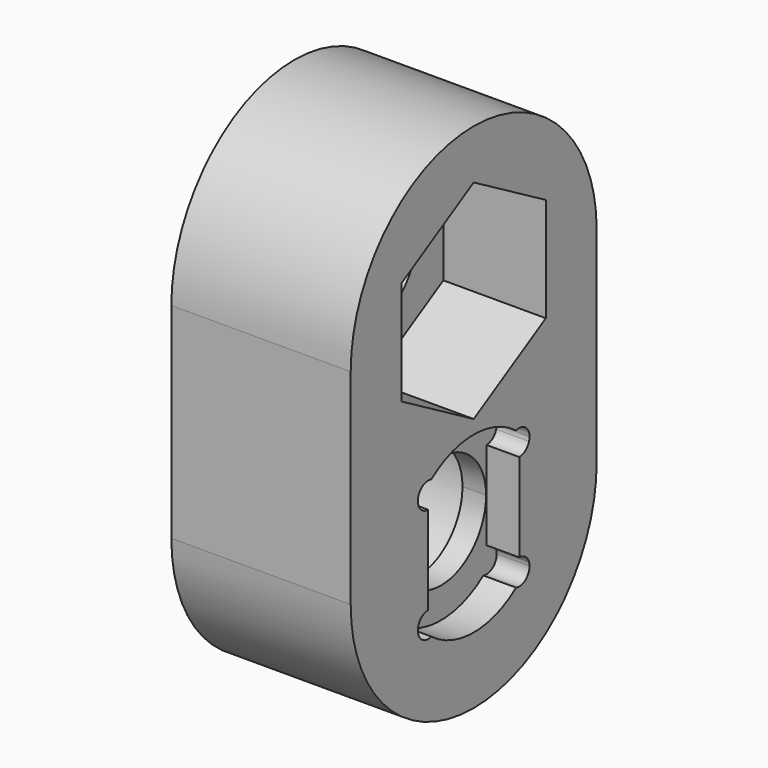
from build123d import *

# Parameters (mm, degrees)
F1_DEPTH = 5.55752
F2_R     = 1.75
F3_DEPTH = 1.016
F4_R     = 1.75
F5_DEPTH = 1.016
F6_DEPTH = 3.175
F7_R     = 2.667
F7_R_2   = 1.75
F8_DEPTH = 3.81


# Not quite as in the source:
# - a feature names something its author has since deleted; it is built from what else it names


with BuildPart() as f1:
    # F0 (on Right) → F1 (new body)
    with BuildSketch(Plane.YZ):
        with BuildLine():
            ThreePointArc((0.636344373, -4.7197957677), (2.2310225415, -4.2076055743), (3.5497579143, -3.175))
            ThreePointArc((3.5497579143, -3.175), (2.2310225415, -2.1423944257), (0.636344373, -1.6302042323))
            ThreePointArc((0.636344373, -1.6302042323), (0, -1.75), (-0.636344373, -1.6302042323))
            ThreePointArc((-0.636344373, -1.6302042323), (-2.2310225415, -2.1423944257), (-3.5497579143, -3.175))
            ThreePointArc((-3.5497579143, -3.175), (-2.2310225415, -4.2076055743), (-0.636344373, -4.7197957677))
            ThreePointArc((-0.636344373, -4.7197957677), (0, -4.6), (0.636344373, -4.7197957677))
        make_face()
        with BuildLine():
            ThreePointArc((3.5497579143, -3.175), (4.4489958596, -1.6993652025), (4.7625, 0))
            ThreePointArc((4.7625, 0), (0, 4.7625), (-4.7625, 0))
            ThreePointArc((-4.7625, 0), (-4.4489958596, -1.6993652025), (-3.5497579143, -3.175))
            ThreePointArc((-3.5497579143, -3.175), (-2.2310225415, -2.1423944257), (-0.636344373, -1.6302042323))
            ThreePointArc((-0.636344373, -1.6302042323), (-0.9871416685, 1.4450091094), (1.75, 0))
            ThreePointArc((1.75, 0), (1.4450091094, -0.9871416685), (0.636344373, -1.6302042323))
            ThreePointArc((0.636344373, -1.6302042323), (2.2310225415, -2.1423944257), (3.5497579143, -3.175))
        make_face()
        with BuildLine():
            Line((4.7625, -6.35), (4.7625, 0))
            ThreePointArc((4.7625, 0), (4.4489958596, -1.6993652025), (3.5497579143, -3.175))
            ThreePointArc((3.5497579143, -3.175), (4.4489958596, -4.6506347975), (4.7625, -6.35))
        make_face()
        with BuildLine():
            ThreePointArc((4.7625, -6.35), (4.4489958596, -4.6506347975), (3.5497579143, -3.175))
            ThreePointArc((3.5497579143, -3.175), (2.2310225415, -4.2076055743), (0.636344373, -4.7197957677))
            ThreePointArc((0.636344373, -4.7197957677), (1.4450091094, -5.3628583315), (1.75, -6.35))
            ThreePointArc((1.75, -6.35), (-0.9871416685, -7.7950091094), (-0.636344373, -4.7197957677))
            ThreePointArc((-0.636344373, -4.7197957677), (-2.2310225415, -4.2076055743), (-3.5497579143, -3.175))
            ThreePointArc((-3.5497579143, -3.175), (-4.4489958596, -4.6506347975), (-4.7625, -6.35))
            ThreePointArc((-4.7625, -6.35), (0, -11.1125), (4.7625, -6.35))
        make_face()
        with BuildLine():
            ThreePointArc((-3.5497579143, -3.175), (-4.4489958596, -1.6993652025), (-4.7625, 0))
            Line((-4.7625, 0), (-4.7625, -6.35))
            ThreePointArc((-4.7625, -6.35), (-4.4489958596, -4.6506347975), (-3.5497579143, -3.175))
        make_face()
    extrude(amount=F1_DEPTH)

    # F2 (on face) → F3 (cut)
    with BuildSketch(Plane.YZ.offset(5.55752)):
        with BuildLine():
            ThreePointArc((1.368425, -4.5847), (1.4846669962, -4.8653330038), (1.7653, -4.981575))
            Line((1.7653, -4.981575), (1.7653, -4.5847))
            Line((1.7653, -4.5847), (1.368425, -4.5847))
        make_face()
        with BuildLine():
            Line((1.7653, -4.5847), (1.7653, -4.981575))
            ThreePointArc((1.7653, -4.981575), (1.9986038099, -4.9057593371), (2.1427708235, -4.7072787218))
            ThreePointArc((2.1427708235, -4.7072787218), (1.9091883092, -4.4408116908), (1.6427212782, -4.2072291765))
            ThreePointArc((1.6427212782, -4.2072291765), (1.4442406629, -4.3513961901), (1.368425, -4.5847))
            Line((1.368425, -4.5847), (1.7653, -4.5847))
        make_face()
        with BuildLine():
            ThreePointArc((1.7653, -7.718425), (1.4846669962, -7.8346669962), (1.368425, -8.1153))
            Line((1.368425, -8.1153), (1.7653, -8.1153))
            Line((1.7653, -8.1153), (1.7653, -7.718425))
        make_face()
        with BuildLine():
            Line((1.7653, -8.1153), (1.368425, -8.1153))
            ThreePointArc((1.368425, -8.1153), (1.4442406629, -8.3486038099), (1.6427212782, -8.4927708235))
            ThreePointArc((1.6427212782, -8.4927708235), (1.9091883092, -8.2591883092), (2.1427708235, -7.9927212782))
            ThreePointArc((2.1427708235, -7.9927212782), (1.9986038099, -7.7942406629), (1.7653, -7.718425))
            Line((1.7653, -7.718425), (1.7653, -8.1153))
        make_face()
        with BuildLine():
            Line((-1.368425, -8.1153), (-1.7653, -8.1153))
            Line((-1.7653, -8.1153), (-1.7653, -7.718425))
            ThreePointArc((-1.7653, -7.718425), (-1.9986038099, -7.7942406629), (-2.1427708235, -7.9927212782))
            ThreePointArc((-2.1427708235, -7.9927212782), (-1.9091883092, -8.2591883092), (-1.6427212782, -8.4927708235))
            ThreePointArc((-1.6427212782, -8.4927708235), (-1.4442406629, -8.3486038099), (-1.368425, -8.1153))
        make_face()
        with BuildLine():
            Line((-1.7653, -7.718425), (-1.7653, -8.1153))
            Line((-1.7653, -8.1153), (-1.368425, -8.1153))
            ThreePointArc((-1.368425, -8.1153), (-1.4846669962, -7.8346669962), (-1.7653, -7.718425))
        make_face()
        with BuildLine():
            Line((-1.7653, -4.5847), (-1.7653, -4.981575))
            ThreePointArc((-1.7653, -4.981575), (-1.4846669962, -4.8653330038), (-1.368425, -4.5847))
            Line((-1.368425, -4.5847), (-1.7653, -4.5847))
        make_face()
        with BuildLine():
            ThreePointArc((-2.1427708235, -4.7072787218), (-1.9986038099, -4.9057593371), (-1.7653, -4.981575))
            Line((-1.7653, -4.981575), (-1.7653, -4.5847))
            Line((-1.7653, -4.5847), (-1.368425, -4.5847))
            ThreePointArc((-1.368425, -4.5847), (-1.4442406629, -4.3513961901), (-1.6427212782, -4.2072291765))
            ThreePointArc((-1.6427212782, -4.2072291765), (-1.9091883092, -4.4408116908), (-2.1427708235, -4.7072787218))
        make_face()
        with BuildLine():
            ThreePointArc((-1.7653, -7.718425), (-1.4846669962, -7.8346669962), (-1.368425, -8.1153))
            Line((-1.368425, -8.1153), (1.368425, -8.1153))
            ThreePointArc((1.368425, -8.1153), (1.4846669962, -7.8346669962), (1.7653, -7.718425))
            Line((1.7653, -7.718425), (1.7653, -4.981575))
            ThreePointArc((1.7653, -4.981575), (1.4846669962, -4.8653330038), (1.368425, -4.5847))
            Line((1.368425, -4.5847), (-1.368425, -4.5847))
            ThreePointArc((-1.368425, -4.5847), (-1.4846669962, -4.8653330038), (-1.7653, -4.981575))
            Line((-1.7653, -4.981575), (-1.7653, -7.718425))
        make_face()
        with Locations((0, -6.35)):
            Circle(F2_R, mode=Mode.SUBTRACT)
        with BuildLine():
            ThreePointArc((-1.6427212782, -4.2072291765), (-2.0459330038, -4.3040669962), (-2.1427708235, -4.7072787218))
            ThreePointArc((-2.1427708235, -4.7072787218), (-1.9091883092, -4.4408116908), (-1.6427212782, -4.2072291765))
        make_face()
        with BuildLine():
            ThreePointArc((1.6427212782, -4.2072291765), (1.9091883092, -4.4408116908), (2.1427708235, -4.7072787218))
            ThreePointArc((2.1427708235, -4.7072787218), (2.1572939405, -4.6467525283), (2.162175, -4.5847))
            ThreePointArc((2.162175, -4.5847), (1.9986038099, -4.2636406629), (1.6427212782, -4.2072291765))
        make_face()
        with BuildLine():
            ThreePointArc((2.1427708235, -7.9927212782), (1.9091883092, -8.2591883092), (1.6427212782, -8.4927708235))
            ThreePointArc((1.6427212782, -8.4927708235), (1.9986038099, -8.4363593371), (2.162175, -8.1153))
            ThreePointArc((2.162175, -8.1153), (2.1572939405, -8.0532474717), (2.1427708235, -7.9927212782))
        make_face()
        with BuildLine():
            ThreePointArc((-2.1427708235, -7.9927212782), (-2.0459330038, -8.3959330038), (-1.6427212782, -8.4927708235))
            ThreePointArc((-1.6427212782, -8.4927708235), (-1.9091883092, -8.2591883092), (-2.1427708235, -7.9927212782))
        make_face()
        with BuildLine():
            ThreePointArc((-1.6427212782, -4.2072291765), (-1.4442406629, -4.3513961901), (-1.368425, -4.5847))
            Line((-1.368425, -4.5847), (1.368425, -4.5847))
            ThreePointArc((1.368425, -4.5847), (1.4442406629, -4.3513961901), (1.6427212782, -4.2072291765))
            ThreePointArc((1.6427212782, -4.2072291765), (0, -3.65), (-1.6427212782, -4.2072291765))
        make_face()
        with BuildLine():
            Line((1.368425, -8.1153), (-1.368425, -8.1153))
            ThreePointArc((-1.368425, -8.1153), (-1.4442406629, -8.3486038099), (-1.6427212782, -8.4927708235))
            ThreePointArc((-1.6427212782, -8.4927708235), (0, -9.05), (1.6427212782, -8.4927708235))
            ThreePointArc((1.6427212782, -8.4927708235), (1.4442406629, -8.3486038099), (1.368425, -8.1153))
        make_face()
    extrude(amount=-F3_DEPTH, mode=Mode.SUBTRACT)

    # F4 (on face) → F5 (cut)
    with BuildSketch(Plane(origin=(0, 0, 0), x_dir=(0, -1, 0), z_dir=(-1, 0, 0))):
        with BuildLine():
            ThreePointArc((1.7653, -1.368425), (1.4846669962, -1.4846669962), (1.368425, -1.7653))
            Line((1.368425, -1.7653), (1.7653, -1.7653))
            Line((1.7653, -1.7653), (1.7653, -1.368425))
        make_face()
        with BuildLine():
            Line((1.7653, -1.7653), (1.368425, -1.7653))
            ThreePointArc((1.368425, -1.7653), (1.4442406629, -1.9986038099), (1.6427212782, -2.1427708235))
            ThreePointArc((1.6427212782, -2.1427708235), (1.9091883092, -1.9091883092), (2.1427708235, -1.6427212782))
            ThreePointArc((2.1427708235, -1.6427212782), (1.9986038099, -1.4442406629), (1.7653, -1.368425))
            Line((1.7653, -1.368425), (1.7653, -1.7653))
        make_face()
        with BuildLine():
            Line((-1.7653, -1.368425), (-1.7653, -1.7653))
            Line((-1.7653, -1.7653), (-1.368425, -1.7653))
            ThreePointArc((-1.368425, -1.7653), (-1.4846669962, -1.4846669962), (-1.7653, -1.368425))
        make_face()
        with BuildLine():
            Line((-1.368425, -1.7653), (-1.7653, -1.7653))
            Line((-1.7653, -1.7653), (-1.7653, -1.368425))
            ThreePointArc((-1.7653, -1.368425), (-1.9986038099, -1.4442406629), (-2.1427708235, -1.6427212782))
            ThreePointArc((-2.1427708235, -1.6427212782), (-1.9091883092, -1.9091883092), (-1.6427212782, -2.1427708235))
            ThreePointArc((-1.6427212782, -2.1427708235), (-1.4442406629, -1.9986038099), (-1.368425, -1.7653))
        make_face()
        with BuildLine():
            Line((-1.7653, 1.7653), (-1.7653, 1.368425))
            ThreePointArc((-1.7653, 1.368425), (-1.4846669962, 1.4846669962), (-1.368425, 1.7653))
            Line((-1.368425, 1.7653), (-1.7653, 1.7653))
        make_face()
        with BuildLine():
            ThreePointArc((-2.1427708235, 1.6427212782), (-1.9986038099, 1.4442406629), (-1.7653, 1.368425))
            Line((-1.7653, 1.368425), (-1.7653, 1.7653))
            Line((-1.7653, 1.7653), (-1.368425, 1.7653))
            ThreePointArc((-1.368425, 1.7653), (-1.4442406629, 1.9986038099), (-1.6427212782, 2.1427708235))
            ThreePointArc((-1.6427212782, 2.1427708235), (-1.9091883092, 1.9091883092), (-2.1427708235, 1.6427212782))
        make_face()
        with BuildLine():
            ThreePointArc((1.368425, 1.7653), (1.4846669962, 1.4846669962), (1.7653, 1.368425))
            Line((1.7653, 1.368425), (1.7653, 1.7653))
            Line((1.7653, 1.7653), (1.368425, 1.7653))
        make_face()
        with BuildLine():
            Line((1.7653, 1.7653), (1.7653, 1.368425))
            ThreePointArc((1.7653, 1.368425), (1.9986038099, 1.4442406629), (2.1427708235, 1.6427212782))
            ThreePointArc((2.1427708235, 1.6427212782), (1.9091883092, 1.9091883092), (1.6427212782, 2.1427708235))
            ThreePointArc((1.6427212782, 2.1427708235), (1.4442406629, 1.9986038099), (1.368425, 1.7653))
            Line((1.368425, 1.7653), (1.7653, 1.7653))
        make_face()
        with BuildLine():
            ThreePointArc((-1.7653, -1.368425), (-1.4846669962, -1.4846669962), (-1.368425, -1.7653))
            Line((-1.368425, -1.7653), (1.368425, -1.7653))
            ThreePointArc((1.368425, -1.7653), (1.4846669962, -1.4846669962), (1.7653, -1.368425))
            Line((1.7653, -1.368425), (1.7653, 1.368425))
            ThreePointArc((1.7653, 1.368425), (1.4846669962, 1.4846669962), (1.368425, 1.7653))
            Line((1.368425, 1.7653), (-1.368425, 1.7653))
            ThreePointArc((-1.368425, 1.7653), (-1.4846669962, 1.4846669962), (-1.7653, 1.368425))
            Line((-1.7653, 1.368425), (-1.7653, -1.368425))
        make_face()
        Circle(F4_R, mode=Mode.SUBTRACT)
        with BuildLine():
            ThreePointArc((-1.6427212782, 2.1427708235), (-2.0459330038, 2.0459330038), (-2.1427708235, 1.6427212782))
            ThreePointArc((-2.1427708235, 1.6427212782), (-1.9091883092, 1.9091883092), (-1.6427212782, 2.1427708235))
        make_face()
        with BuildLine():
            ThreePointArc((1.6427212782, 2.1427708235), (1.9091883092, 1.9091883092), (2.1427708235, 1.6427212782))
            ThreePointArc((2.1427708235, 1.6427212782), (2.1572939405, 1.7032474717), (2.162175, 1.7653))
            ThreePointArc((2.162175, 1.7653), (1.9986038099, 2.0863593371), (1.6427212782, 2.1427708235))
        make_face()
        with BuildLine():
            ThreePointArc((2.1427708235, -1.6427212782), (1.9091883092, -1.9091883092), (1.6427212782, -2.1427708235))
            ThreePointArc((1.6427212782, -2.1427708235), (1.9986038099, -2.0863593371), (2.162175, -1.7653))
            ThreePointArc((2.162175, -1.7653), (2.1572939405, -1.7032474717), (2.1427708235, -1.6427212782))
        make_face()
        with BuildLine():
            ThreePointArc((-2.1427708235, -1.6427212782), (-2.0459330038, -2.0459330038), (-1.6427212782, -2.1427708235))
            ThreePointArc((-1.6427212782, -2.1427708235), (-1.9091883092, -1.9091883092), (-2.1427708235, -1.6427212782))
        make_face()
        with BuildLine():
            Line((1.368425, -1.7653), (-1.368425, -1.7653))
            ThreePointArc((-1.368425, -1.7653), (-1.4442406629, -1.9986038099), (-1.6427212782, -2.1427708235))
            ThreePointArc((-1.6427212782, -2.1427708235), (0, -2.7), (1.6427212782, -2.1427708235))
            ThreePointArc((1.6427212782, -2.1427708235), (1.4442406629, -1.9986038099), (1.368425, -1.7653))
        make_face()
        with BuildLine():
            ThreePointArc((-1.6427212782, 2.1427708235), (-1.4442406629, 1.9986038099), (-1.368425, 1.7653))
            Line((-1.368425, 1.7653), (1.368425, 1.7653))
            ThreePointArc((1.368425, 1.7653), (1.4442406629, 1.9986038099), (1.6427212782, 2.1427708235))
            ThreePointArc((1.6427212782, 2.1427708235), (0, 2.7), (-1.6427212782, 2.1427708235))
        make_face()
    extrude(amount=-F5_DEPTH, mode=Mode.SUBTRACT)

    # F2 (on face) → F6 (cut)
    with BuildSketch(Plane.YZ.offset(5.55752)):
        Polygon((-2.794, -1.6131166521), (0, -3.2262333042), (2.794, -1.6131166521), (2.794, 1.6131166521), (0, 3.2262333042), (-2.794, 1.6131166521), align=None)
        Circle(F2_R, mode=Mode.SUBTRACT)
    extrude(amount=-F6_DEPTH, mode=Mode.SUBTRACT)

    # F7 (on face) → F8 (cut)
    with BuildSketch(Plane(origin=(0, 0, 0), x_dir=(0, -1, 0), z_dir=(-1, 0, 0))):
        with Locations((0, -6.35)):
            Circle(F7_R)
        with Locations((0, -6.35)):
            Circle(F7_R_2, mode=Mode.SUBTRACT)
    extrude(amount=-F8_DEPTH, mode=Mode.SUBTRACT)


solid = f1.part
